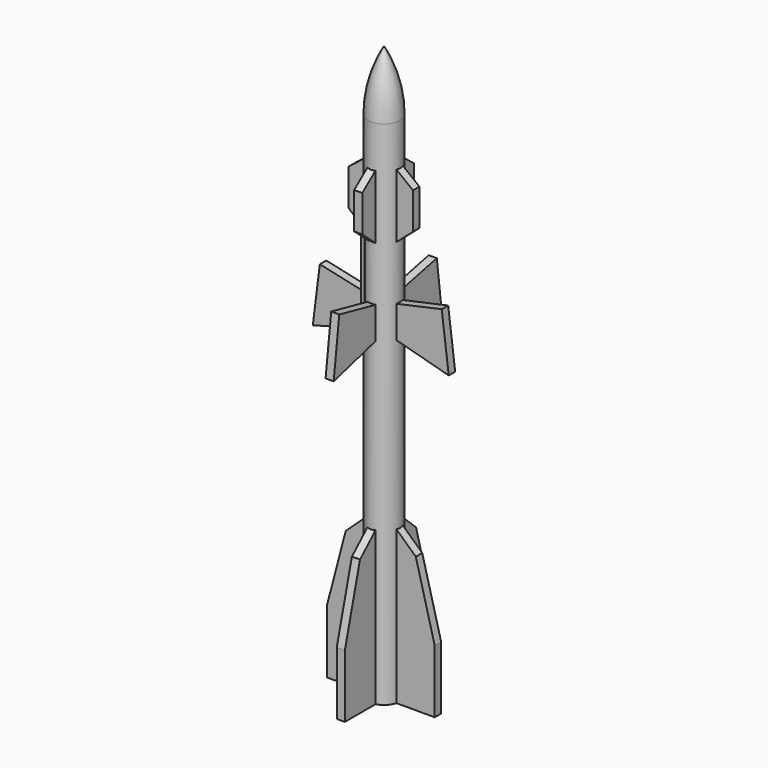
from build123d import *

# Parameters (mm, degrees)
F4_DEPTH     = 0.2
F5_COUNT     = 4
F8_DEPTH     = 6.0416666667
F9_T4_ANGLE  = 67.1804235359
F9_S7_R      = 0.25
F9_T8_DEPTH  = 2
F9_T12_ANGLE = 67.1804235359
F9_S13_R     = 0.25
F9_T14_DEPTH = 2


# Not quite as in the source:
# - a fillet or chamfer that OpenCascade refuses, or shapes differently, is made with other operations: its cross-section is extruded or revolved along the edge and cut away or added


with BuildPart() as f2:
    # F1 (on Front) → F2 (revolve)
    with BuildSketch(Plane.XZ):
        with BuildLine():
            Line((0, 28.3333333333), (0, 0))
            Line((0, 0), (0.7986111111, 0))
            Line((0.7986111111, 0), (0.7986111111, 25.3472222222))
            ThreePointArc((0.7986111111, 25.3472222222), (0.5955105226, 26.8927511992), (0, 28.3333333333))
        make_face()
    revolve(axis=Axis((0, 0, 14.1666666667), (0, 0, 1)))

    # F3 (on Front) → F4 (join, symmetric)
    with BuildSketch(Plane.XZ):
        Polygon((0, 23.8888888889), (0, 0), (0.7986111111, 0), (2.6736111111, 0), (2.6736111111, 3.125), (1.7361111111, 6.7013888889), (0.4, 7.9385288066), (0.4, 15.9410660661), (3.3680555556, 15.1388888889), (3.0208333333, 17.9166666667), (0.4, 17.343359375), (0.4, 19.7922705314), (1.5972222222, 20.8333333333), (1.5972222222, 22.6388888889), align=None)
    extrude(amount=F4_DEPTH, both=True)

    # F5: F2 ×4 about axis
    f5_axis = Axis((0, 0, 0), (0, 0, 1))


with BuildPart() as f2_1:
    add(f2.part)
    for i in range(1, F5_COUNT):
        add(f2.part.rotate(f5_axis, i * 360 / F5_COUNT))

    # F7 (on offset) → F8 (join)
    with BuildSketch(Plane.XY.offset(15.4166666667)):
        with BuildLine():
            Line((-0.4086259328, -0.7035839656), (-0.1424359704, -0.4373940032))
            Line((-0.1424359704, -0.4373940032), (-0.4373940032, -0.1424359704))
            Line((-0.4373940032, -0.1424359704), (-0.7035839656, -0.4086259328))
            ThreePointArc((-0.7035839656, -0.4086259328), (-0.6354140103, -0.6354140103), (-0.4086259328, -0.7035839656))
        make_face()
    extrude(amount=F8_DEPTH)

    # F9: chamfer of 0.1 on 2 edges, made by hand


with BuildPart() as f9_tool2:
    # F9_s3 → F9_t4 (revolve)
    with BuildSketch(Plane(origin=(0, 0, 0), x_dir=(0, 0, 1), z_dir=(-0.197824804, 0.9802373932, 0))):
        Polygon((15.3166666667, -0.7986111111), (15.4166666667, -0.8986111111), (15.4166666667, -0.7986111111), align=None)
    revolve(axis=Axis((0, 0, 15.4166666667), (0, 0, 1)), revolution_arc=F9_T4_ANGLE)

    split(bisect_by=Plane(origin=(0.1474790164, -0.1474790164, 0), x_dir=(0, 0, 1), z_dir=(-0.7071067812, 0.7071067812, 0)), keep=Keep.TOP)

    split(bisect_by=Plane(origin=(-0.1474790164, 0.1474790164, 0), x_dir=(0, 0, 1), z_dir=(0.7071067812, -0.7071067812, 0)), keep=Keep.TOP)

    # F9_s7 → F9_t8 (intersect, symmetric)
    with BuildSketch(Plane.XY.offset(15.4)):
        with Locations((-0.458637315, -0.458637315)):
            Circle(F9_S7_R)
    extrude(amount=F9_T8_DEPTH, both=True, mode=Mode.INTERSECT)


with BuildPart() as f2_2:
    add(f2_1.part)

    # F9_t1: union F9_tool2
    add(f9_tool2.part)


with BuildPart() as f9_tool10:
    # F9_s11 → F9_t12 (revolve)
    with BuildSketch(Plane(origin=(0, 0, 0), x_dir=(0, 0, 1), z_dir=(-0.197824804, 0.9802373932, 0))):
        Polygon((21.5583333333, -0.7986111111), (21.4583333333, -0.8986111111), (21.4583333333, -0.7986111111), align=None)
    revolve(axis=Axis((0, 0, 21.4583333333), (0, 0, 1)), revolution_arc=F9_T12_ANGLE)

    # F9_s13 → F9_t14 (intersect, symmetric)
    with BuildSketch(Plane.XY.offset(21.5)):
        with Locations((-0.458637315, -0.458637315)):
            Circle(F9_S13_R)
    extrude(amount=F9_T14_DEPTH, both=True, mode=Mode.INTERSECT)

    split(bisect_by=Plane(origin=(-0.1474790164, 0.1474790164, 0), x_dir=(0, 0, 1), z_dir=(0.7071067812, -0.7071067812, 0)), keep=Keep.TOP)

    split(bisect_by=Plane(origin=(0.1474790164, -0.1474790164, 0), x_dir=(0, 0, 1), z_dir=(-0.7071067812, 0.7071067812, 0)), keep=Keep.TOP)


with BuildPart() as f2_3:
    add(f2_2.part)

    # F9_t9: union F9_tool10
    add(f9_tool10.part)


solid = f2_3.part
